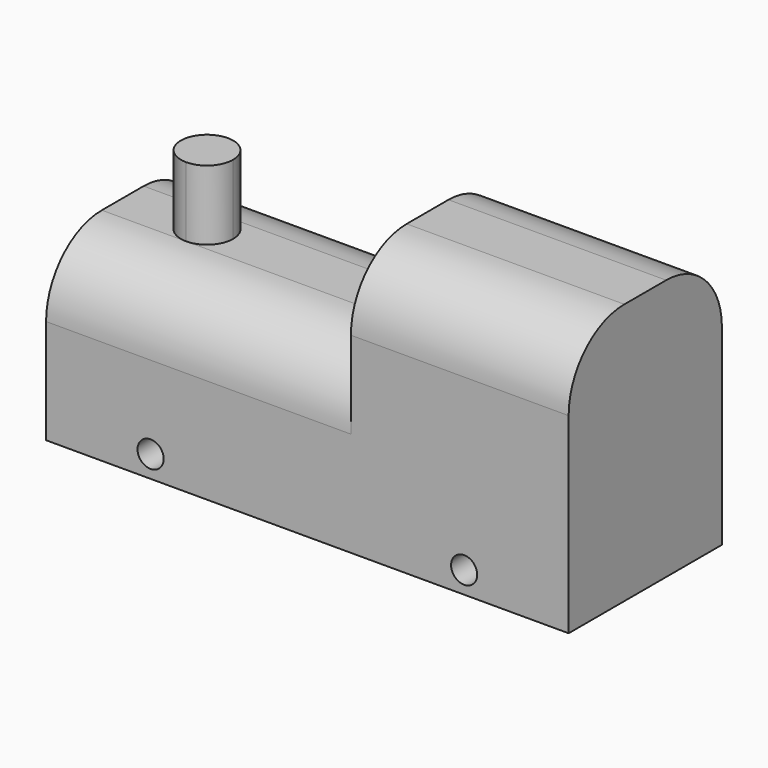
from build123d import *

# Parameters (mm, degrees)
F0_W     = 35
F0_H     = 20
F0_W_2   = 25
F0_H_2   = 10
F1_DEPTH = 11
F2_R     = 8
F3_R     = 8
F5_DEPTH = 8
F6_R     = 1.5
F7_DEPTH = 12.5


# Not quite as in the source:
# - a pattern or mirror of a feature is missing from the dataset's text; its kind, count and spacing are read off the source's solid


with BuildPart() as f1:
    # F0 (on Front) → F1 (new body, symmetric)
    with BuildSketch(Plane.XZ):
        with Locations((17.5, 10)):
            Rectangle(F0_W, F0_H)
        with Locations((47.5, 10)):
            Rectangle(F0_W_2, F0_H)
        with Locations((47.5, 25)):
            Rectangle(F0_W_2, F0_H_2)
    extrude(amount=F1_DEPTH, both=True)

    # F2
    f2_edges = [f1.edges().sort_by_distance(p)[0] for p in [
        (17.5, -11, 20),
        (17.5, 11, 20),
    ]]
    fillet(f2_edges, radius=F2_R)

    # F3
    f3_edges = [f1.edges().sort_by_distance(p)[0] for p in [
        (47.5, -11, 30),
        (47.5, 11, 30),
    ]]
    fillet(f3_edges, radius=F3_R)

    # F4 (on face) → F5 (join)
    with BuildSketch(Plane.XY.offset(20)):
        with BuildLine():
            ThreePointArc((9.6768597141, -3), (11.7981800577, -2.1213203436), (12.6768597141, 0))
            ThreePointArc((12.6768597141, 0), (11.7981800577, 2.1213203436), (9.6768597141, 3))
            ThreePointArc((9.6768597141, 3), (6.6768597141, 0), (9.6768597141, -3))
        make_face()
    extrude(amount=F5_DEPTH)

    # F6 (on Front) → F7 (cut, symmetric)
    with BuildSketch(Plane.XZ):
        with Locations((12, 2.5)):
            Circle(F6_R)
    f7 = extrude(amount=F7_DEPTH, both=True, mode=Mode.SUBTRACT)

    # F7_copies: F7 across plane
    add(f7.mirror(Plane(origin=(30, 0, 0), x_dir=(0, 0, 1), z_dir=(1, 0, 0))), mode=Mode.SUBTRACT)


solid = f1.part
